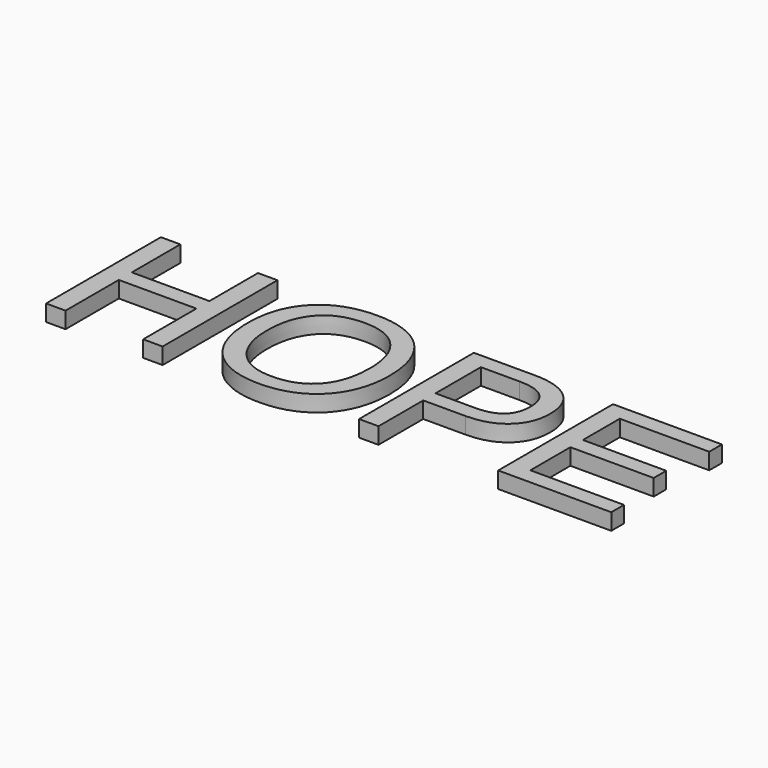
from build123d import *

# Parameters (mm, degrees)
F0_TEXT_SIZE = 105.7455316186
F1_DEPTH     = 8.3007961512


# Not quite as in the source:
# - Text() gives the source's letters only with a copy of the font that has no kerning and outlines rounded to 1/6400 em; it was checked with that copy


with BuildPart() as f1:
    # F0 (on Top) → F1 (new body)
    with BuildSketch(Plane.XY):
        with Locations((-75.7218897343, 0)):
            Text('HOPE', F0_TEXT_SIZE, font='Arimo', text_align=(TextAlign.LEFT, TextAlign.BOTTOM))
    extrude(amount=F1_DEPTH)


solid = f1.part
